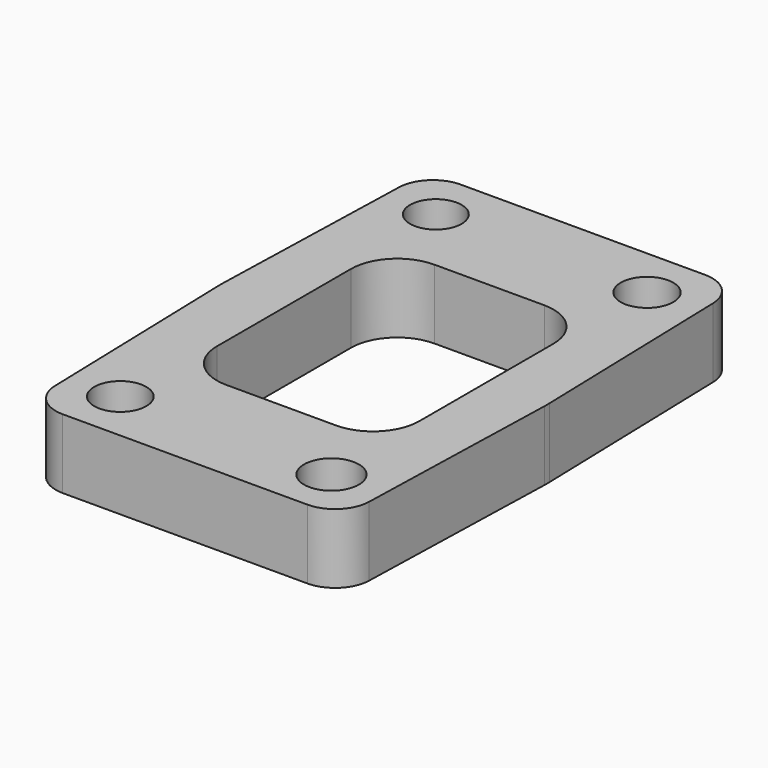
from build123d import *

# Parameters (mm, degrees)
F0_R        = 5.7271899427
F0_R_2      = 6.0263161758
F0_R_3      = 5.6540098822
F0_R_4      = 5.7746792183
F1_DEPTH    = 15.24
F2_T1_DEPTH = 18.788208103
F2_T3_DEPTH = 18.873984206


# Not quite as in the source:
# - a fillet or chamfer that OpenCascade refuses, or shapes differently, is made with other operations: its cross-section is extruded or revolved along the edge and cut away or added


with BuildPart() as f1:
    # F0 (on Top) → F1 (new body)
    with BuildSketch(Plane.XY):
        with BuildLine():
            Line((-126.2685924224, 95.313180417), (-179.9737472962, 95.313180417))
            ThreePointArc((-179.9737472962, 95.313180417), (-185.2842850362, 93.1578477365), (-187.5906297205, 87.9111302629))
            Line((-187.5906297205, 87.9111302629), (-188.941179568, 40.7122925946))
            Line((-188.941179568, 40.7122925946), (-187.5906297205, -6.4865450738))
            ThreePointArc((-187.5906297205, -6.4865450738), (-185.2842850362, -11.7332625474), (-179.9737472962, -13.8885952279))
            Line((-179.9737472962, -13.8885952279), (-126.2685924224, -13.8885952279))
            ThreePointArc((-126.2685924224, -13.8885952279), (-120.9562110346, -11.7314702942), (-118.6515646464, -6.4814046742))
            Line((-118.6515646464, -6.4814046742), (-117.3330366223, 40.7122925946))
            Line((-117.3330366223, 40.7122925946), (-118.6515646464, 87.9059898633))
            ThreePointArc((-118.6515646464, 87.9059898633), (-120.9562110346, 93.1560554834), (-126.2685924224, 95.313180417))
        make_face()
        with Locations((-176.378503075, -2.5813533248)):
            Circle(F0_R, mode=Mode.SUBTRACT)
        with Locations((-130.0195976365, -2.5813533248)):
            Circle(F0_R_2, mode=Mode.SUBTRACT)
        with BuildLine():
            Line((-130.635044248, 59.1215779044), (-130.6350442799, 22.2915779044))
            ThreePointArc((-130.6350442799, 22.2915779044), (-133.610839383, 15.1073730075), (-140.7950442799, 12.1315779044))
            Line((-140.7950442799, 12.1315779044), (-164.9250442799, 12.1315779044))
            ThreePointArc((-164.9250442799, 12.1315779044), (-172.1092491767, 15.1073730075), (-175.0850442799, 22.2915779044))
            Line((-175.0850442799, 22.2915779044), (-175.0850442799, 59.1215779044))
            ThreePointArc((-175.0850442799, 59.1215779044), (-172.1092491767, 66.3057828012), (-164.9250442799, 69.2815779044))
            Line((-164.9250442799, 69.2815779044), (-140.7950442799, 69.2815779044))
            ThreePointArc((-140.7950442799, 69.2815779044), (-133.6108393717, 66.3057828031), (-130.635044248, 59.1215779044))
        make_face(mode=Mode.SUBTRACT)
        with Locations((-176.378503075, 84.005938514)):
            Circle(F0_R_3, mode=Mode.SUBTRACT)
        with Locations((-130.0195976365, 84.005938514)):
            Circle(F0_R_4, mode=Mode.SUBTRACT)
    extrude(amount=F1_DEPTH)

    # F2: fillet of radius 25.4 on 2 edges, made by hand

    # F2_s2 → F2_t1 (cut)
    with BuildSketch(Plane.XY.offset(-1.7741040515)):
        with BuildLine():
            ThreePointArc((-117.3528553153, 40.0029277737), (-117.3429479018, 40.7122925946), (-117.3528553153, 41.4216574155))
            Line((-117.3528553153, 41.4216574155), (-117.3330366223, 40.7122925946))
            Line((-117.3330366223, 40.7122925946), (-117.3528553153, 40.0029277737))
        make_face()
    extrude(amount=F2_T1_DEPTH, mode=Mode.SUBTRACT)

    # F2_s4 → F2_t3 (cut)
    with BuildSketch(Plane.XY.offset(-1.816992103)):
        with BuildLine():
            ThreePointArc((-188.9203914761, 41.4387920809), (-188.9307833954, 40.7122925946), (-188.9203914761, 39.9857931082))
            Line((-188.9203914761, 39.9857931082), (-188.941179568, 40.7122925946))
            Line((-188.941179568, 40.7122925946), (-188.9203914761, 41.4387920809))
        make_face()
    extrude(amount=F2_T3_DEPTH, mode=Mode.SUBTRACT)


solid = f1.part
